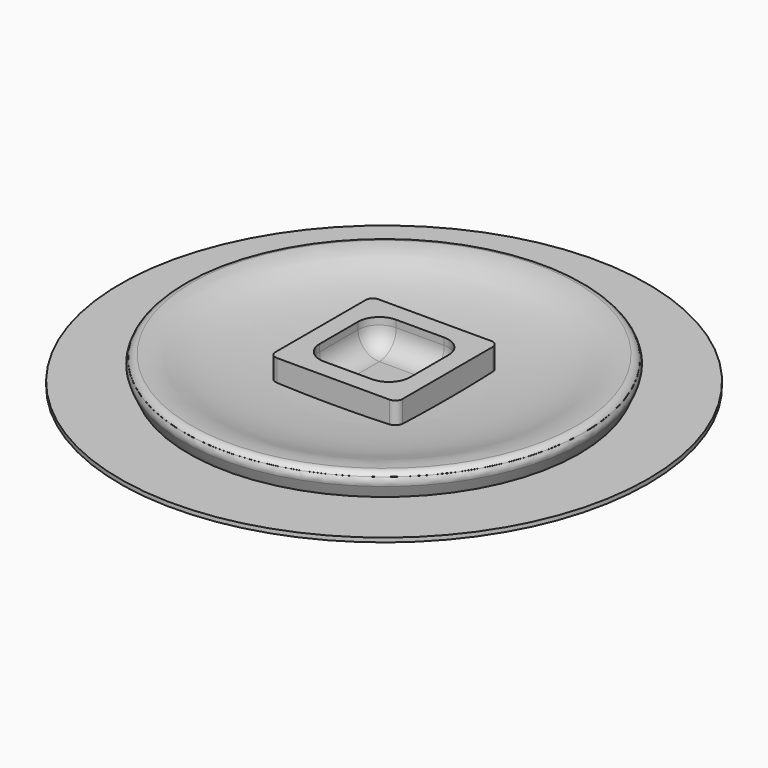
from build123d import *

# Parameters (mm, degrees)
F0_R      = 18.7
F0_R_2    = 13.7
F1_DEPTH  = 0.3
F2_DEPTH  = 2
F2_TAPER  = -24
F4_R      = 0.6
F8_W      = 9
F8_H      = 9
F9_DEPTH  = 2
F10_R     = 0.5
F11_W     = 6.4
F11_H     = 6.4
F12_DEPTH = 2
F13_R     = 1.5


# Not quite as in the source:
# - a fillet or chamfer that OpenCascade refuses, or shapes differently, is made with other operations: its cross-section is extruded or revolved along the edge and cut away or added


with BuildPart() as f1:
    # F0 (on Top) → F1 (new body)
    with BuildSketch(Plane.XY):
        Circle(F0_R)
        Circle(F0_R_2, mode=Mode.SUBTRACT)
        Circle(F0_R_2)
    extrude(amount=F1_DEPTH)

    # F0 (on Top) → F2 (join)
    with BuildSketch(Plane.XY):
        Circle(F0_R_2)
    extrude(amount=F2_DEPTH, taper=F2_TAPER)

    # F3: chamfer of 0.6 on 1 edges, made by hand

    # F3_s1 → F3_t2 (revolve, cut)
    with BuildSketch(Plane.XZ):
        Polygon((14.3464153848, 1.4518727254), (13.9904573706, 2), (14.5904573706, 2), align=None)
    revolve(axis=Axis((0, 0, 2), (0, 0, -1)), mode=Mode.SUBTRACT)

    # F4
    f4_edges = [f1.edges().sort_by_distance(p)[0] for p in [
        (-14.346415, 0, 1.451873),
        (-13.990457, 0, 2),
    ]]
    fillet(f4_edges, radius=F4_R)


with BuildPart() as f6:
    # F5 (on Front) → F6 (revolve)
    with BuildSketch(Plane.XZ):
        with BuildLine():
            Line((0, 2), (-13.6646839508, 2))
            add(Edge.make_bspline(
                [(-13.6646839508, 2), (-11.1315483197, 2), (-12.2314980254, 0.6), (0, 0.6)],
                knots=[0, 0, 0, 0, 13.7362144522, 13.7362144522, 13.7362144522, 13.7362144522], degree=3))
            Line((0, 0.6), (0, 2))
        make_face()
    revolve(axis=Axis((0, 0, 1.3), (0, 0, -1)))


with BuildPart() as f1_1:
    add(f1.part)

    # F7: cut F6
    add(f6.part, mode=Mode.SUBTRACT)

    # F8 (on face) → F9 (join)
    with BuildSketch(Plane.XY.offset(0.3)):
        Rectangle(F8_W, F8_H)
    extrude(amount=F9_DEPTH)

    # F10
    f10_edges = [f1_1.edges().sort_by_distance(p)[0] for p in [
        (-4.5, 4.5, 1.538289),
        (-4.5, -4.5, 1.538289),
        (4.5, -4.5, 1.538289),
        (4.5, 4.5, 1.538289),
    ]]
    fillet(f10_edges, radius=F10_R)

    # F11 (on face) → F12 (cut, through all)
    with BuildSketch(Plane.XY.offset(2.3)):
        Rectangle(F11_W, F11_H)
    extrude(amount=-F12_DEPTH, mode=Mode.SUBTRACT)

    # F13
    f13_edges = [f1_1.edges().sort_by_distance(p)[0] for p in [
        (-3.2, 3.2, 1.3),
        (3.2, 3.2, 1.3),
        (3.2, -3.2, 1.3),
        (-3.2, -3.2, 1.3),
        (0, -3.2, 0.3),
        (3.2, 0, 0.3),
        (0, 3.2, 0.3),
        (-3.2, 0, 0.3),
    ]]
    fillet(f13_edges, radius=F13_R)


solid = f1_1.part
